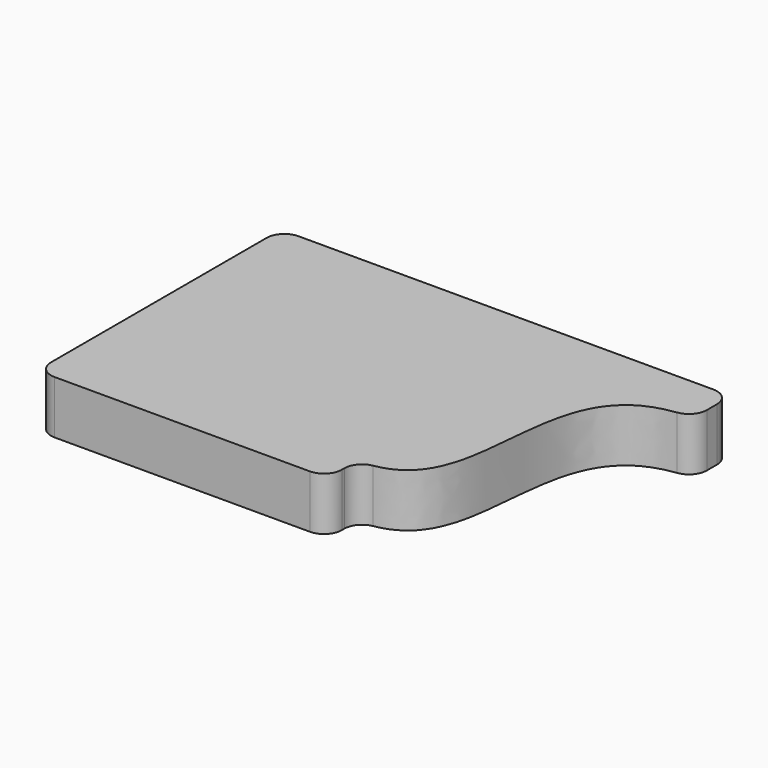
from build123d import *

# Parameters (mm, degrees)
F1_DEPTH    = 15
F2_DEPTH    = 10
F3_T1_DEPTH = 10
F3_T3_DEPTH = 15
F3_T5_DEPTH = 10
F3_T7_DEPTH = 15


# Not quite as in the source:
# - a fillet or chamfer that OpenCascade refuses, or shapes differently, is made with other operations: its cross-section is extruded or revolved along the edge and cut away or added


with BuildPart() as f1:
    # F0 (on Top) → F1 (new body)
    with BuildSketch(Plane.XY):
        with BuildLine():
            Line((49.4806755117, 19.463416189), (49.4806755117, 32.7418245673))
            Line((49.4806755117, 32.7418245673), (-77.5193244883, 32.7418245673))
            Line((-77.5193244883, 32.7418245673), (-77.5193244883, -53.2581754327))
            Line((-77.5193244883, -53.2581754327), (4.4806755117, -53.2581754327))
            Line((4.4806755117, -53.2581754327), (4.4806755117, -42.7682958543))
            add(Edge.make_bspline(
                [(49.4806755117, 19.463416189), (7.0367345721, 19.1974722368), (40.0757081807, -42.7682958543), (4.4806755117, -42.7682958543)],
                knots=[0, 0, 0, 0, 76.7970441088, 76.7970441088, 76.7970441088, 76.7970441088], degree=3))
        make_face()
        with BuildLine():
            Line((-75.5193244883, 30.7418245673), (47.4806755117, 30.7418245673))
            Line((47.4806755117, 30.7418245673), (47.4806755117, 21.7418245673))
            add(Edge.make_bspline(
                [(47.4806755117, 21.7418245673), (7.0367345721, 21.7418245681), (35.4659482837, -40.9756116569), (2.4806755117, -40.2581754327)],
                knots=[0, 0, 0, 0, 76.6093989012, 76.6093989012, 76.6093989012, 76.6093989012], degree=3))
            Line((2.4806755117, -40.2581754327), (2.4806755117, -51.2581754327))
            Line((2.4806755117, -51.2581754327), (-75.5193244883, -51.2581754327))
            Line((-75.5193244883, -51.2581754327), (-75.5193244883, 30.7418245673))
        make_face(mode=Mode.SUBTRACT)
        with BuildLine():
            Line((47.4806755117, 21.7418245673), (47.4806755117, 30.7418245673))
            Line((47.4806755117, 30.7418245673), (-75.5193244883, 30.7418245673))
            Line((-75.5193244883, 30.7418245673), (-75.5193244883, -51.2581754327))
            Line((-75.5193244883, -51.2581754327), (2.4806755117, -51.2581754327))
            Line((2.4806755117, -51.2581754327), (2.4806755117, -40.2581754327))
            add(Edge.make_bspline(
                [(47.4806755117, 21.7418245673), (7.0367345721, 21.7418245681), (35.4659482837, -40.9756116569), (2.4806755117, -40.2581754327)],
                knots=[0, 0, 0, 0, 76.6093989012, 76.6093989012, 76.6093989012, 76.6093989012], degree=3))
        make_face()
    extrude(amount=F1_DEPTH)

    # F0 (on Top) → F2 (cut)
    with BuildSketch(Plane.XY):
        with BuildLine():
            Line((47.4806755117, 21.7418245673), (47.4806755117, 30.7418245673))
            Line((47.4806755117, 30.7418245673), (-75.5193244883, 30.7418245673))
            Line((-75.5193244883, 30.7418245673), (-75.5193244883, -51.2581754327))
            Line((-75.5193244883, -51.2581754327), (2.4806755117, -51.2581754327))
            Line((2.4806755117, -51.2581754327), (2.4806755117, -40.2581754327))
            add(Edge.make_bspline(
                [(47.4806755117, 21.7418245673), (7.0367345721, 21.7418245681), (35.4659482837, -40.9756116569), (2.4806755117, -40.2581754327)],
                knots=[0, 0, 0, 0, 76.6093989012, 76.6093989012, 76.6093989012, 76.6093989012], degree=3))
        make_face()
    extrude(amount=F2_DEPTH, mode=Mode.SUBTRACT)

    # F3: fillet of radius 5 on 12 edges, made by hand

    # F3_s2 → F3_t1 (join)
    with BuildSketch(Plane.XY):
        with BuildLine():
            ThreePointArc((-2.5193244883, -51.2581754327), (1.0162094176, -49.7937093386), (2.4806755117, -46.2581754327))
            Line((2.4806755117, -46.2581754327), (2.5806755117, -46.2581754327))
            Line((2.5806755117, -46.2581754327), (2.5806755117, -51.3581754327))
            Line((2.5806755117, -51.3581754327), (-2.5193244883, -51.3581754327))
            Line((-2.5193244883, -51.3581754327), (-2.5193244883, -51.2581754327))
        make_face()
        with BuildLine():
            ThreePointArc((-75.5193244883, -46.2581754327), (-74.0548583942, -49.7937093386), (-70.5193244883, -51.2581754327))
            Line((-70.5193244883, -51.2581754327), (-70.5193244883, -51.3581754327))
            Line((-70.5193244883, -51.3581754327), (-75.6193244883, -51.3581754327))
            Line((-75.6193244883, -51.3581754327), (-75.6193244883, -46.2581754327))
            Line((-75.6193244883, -46.2581754327), (-75.5193244883, -46.2581754327))
        make_face()
        with BuildLine():
            ThreePointArc((47.4806755117, 25.7418245673), (46.0162094176, 29.2773584733), (42.4806755117, 30.7418245673))
            Line((42.4806755117, 30.7418245673), (42.4806755117, 30.8418245673))
            Line((42.4806755117, 30.8418245673), (47.5806755117, 30.8418245673))
            Line((47.5806755117, 30.8418245673), (47.5806755117, 25.7418245673))
            Line((47.5806755117, 25.7418245673), (47.4806755117, 25.7418245673))
        make_face()
        with BuildLine():
            ThreePointArc((47.4806755117, 26.4306458763), (46.2382757051, 23.1320945599), (43.128499197, 21.4727910505))
            Line((43.128499197, 21.4727910505), (43.1414556707, 21.373633954))
            ThreePointArc((43.1414556707, 21.373633954), (45.3063470559, 21.5780729271), (47.4806755117, 21.6418245673))
            Line((47.4806755117, 21.6418245673), (47.5806755117, 21.7418245673))
            Line((47.5806755117, 21.7418245673), (47.5806755117, 26.4306458763))
            Line((47.5806755117, 26.4306458763), (47.4806755117, 26.4306458763))
        make_face()
        with BuildLine():
            ThreePointArc((-70.5193244883, 30.7418245673), (-74.0548583942, 29.2773584733), (-75.5193244883, 25.7418245673))
            Line((-75.5193244883, 25.7418245673), (-75.6193244883, 25.7418245673))
            Line((-75.6193244883, 25.7418245673), (-75.6193244883, 30.8418245673))
            Line((-75.6193244883, 30.8418245673), (-70.5193244883, 30.8418245673))
            Line((-70.5193244883, 30.8418245673), (-70.5193244883, 30.7418245673))
        make_face()
    extrude(amount=F3_T1_DEPTH)

    # F3_s4 → F3_t3 (join)
    with BuildSketch(Plane.XY):
        with BuildLine():
            ThreePointArc((8.6534072199, -42.4428158907), (5.6638481997, -44.1440694712), (4.4806755117, -47.3739037193))
            Line((4.4806755117, -47.3739037193), (4.3806755117, -47.3739037193))
            Line((4.3806755117, -47.3739037193), (4.3806755117, -42.7682958543))
            Line((4.3806755117, -42.7682958543), (4.4806755117, -42.6682958543))
            ThreePointArc((4.4806755117, -42.6682958543), (6.5660460923, -42.592345805), (8.6368618541, -42.3441941341))
            Line((8.6368618541, -42.3441941341), (8.6534072199, -42.4428158907))
        make_face()
    extrude(amount=F3_T3_DEPTH)

    # F3_s6 → F3_t5 (cut)
    with BuildSketch(Plane.XY):
        with BuildLine():
            ThreePointArc((2.4806755117, -44.8983401385), (3.654280904, -41.6798460331), (6.6241572343, -39.9722487426))
            Line((6.6241572343, -39.9722487426), (6.6070268687, -39.8737269147))
            ThreePointArc((6.6070268687, -39.8737269147), (4.5524483639, -40.1156981702), (2.4828500173, -40.1581990778))
            Line((2.4828500173, -40.1581990778), (2.3806755117, -40.2581754327))
            Line((2.3806755117, -40.2581754327), (2.3806755117, -44.8983401385))
            Line((2.3806755117, -44.8983401385), (2.4806755117, -44.8983401385))
        make_face()
    extrude(amount=F3_T5_DEPTH, mode=Mode.SUBTRACT)

    # F3_s8 → F3_t7 (cut)
    with BuildSketch(Plane.XY):
        with BuildLine():
            ThreePointArc((-77.5193244883, 27.7418245673), (-76.0548583942, 31.2773584733), (-72.5193244883, 32.7418245673))
            Line((-72.5193244883, 32.7418245673), (-72.5193244883, 32.8418245673))
            Line((-72.5193244883, 32.8418245673), (-77.6193244883, 32.8418245673))
            Line((-77.6193244883, 32.8418245673), (-77.6193244883, 27.7418245673))
            Line((-77.6193244883, 27.7418245673), (-77.5193244883, 27.7418245673))
        make_face()
        with BuildLine():
            ThreePointArc((-72.5193244883, -53.2581754327), (-76.0548583942, -51.7937093386), (-77.5193244883, -48.2581754327))
            Line((-77.5193244883, -48.2581754327), (-77.6193244883, -48.2581754327))
            Line((-77.6193244883, -48.2581754327), (-77.6193244883, -53.3581754327))
            Line((-77.6193244883, -53.3581754327), (-72.5193244883, -53.3581754327))
            Line((-72.5193244883, -53.3581754327), (-72.5193244883, -53.2581754327))
        make_face()
        with BuildLine():
            ThreePointArc((4.4806755117, -48.2581754327), (3.0162094176, -51.7937093386), (-0.5193244883, -53.2581754327))
            Line((-0.5193244883, -53.2581754327), (-0.5193244883, -53.3581754327))
            Line((-0.5193244883, -53.3581754327), (4.5806755117, -53.3581754327))
            Line((4.5806755117, -53.3581754327), (4.5806755117, -48.2581754327))
            Line((4.5806755117, -48.2581754327), (4.4806755117, -48.2581754327))
        make_face()
        with BuildLine():
            ThreePointArc((45.1004422697, 19.1903117186), (48.2289306918, 20.8425854223), (49.4806755117, 24.1517519495))
            Line((49.4806755117, 24.1517519495), (49.5806755117, 24.1517519495))
            Line((49.5806755117, 24.1517519495), (49.5806755117, 19.463416189))
            Line((49.5806755117, 19.463416189), (49.4813020764, 19.3634181519))
            ThreePointArc((49.4813020764, 19.3634181519), (47.2927078664, 19.2915430386), (45.1128376048, 19.0910829139))
            Line((45.1128376048, 19.0910829139), (45.1004422697, 19.1903117186))
        make_face()
        with BuildLine():
            ThreePointArc((44.4806755117, 32.7418245673), (48.0162094176, 31.2773584733), (49.4806755117, 27.7418245673))
            Line((49.4806755117, 27.7418245673), (49.5806755117, 27.7418245673))
            Line((49.5806755117, 27.7418245673), (49.5806755117, 32.8418245673))
            Line((49.5806755117, 32.8418245673), (44.4806755117, 32.8418245673))
            Line((44.4806755117, 32.8418245673), (44.4806755117, 32.7418245673))
        make_face()
    extrude(amount=F3_T7_DEPTH, mode=Mode.SUBTRACT)


solid = f1.part
